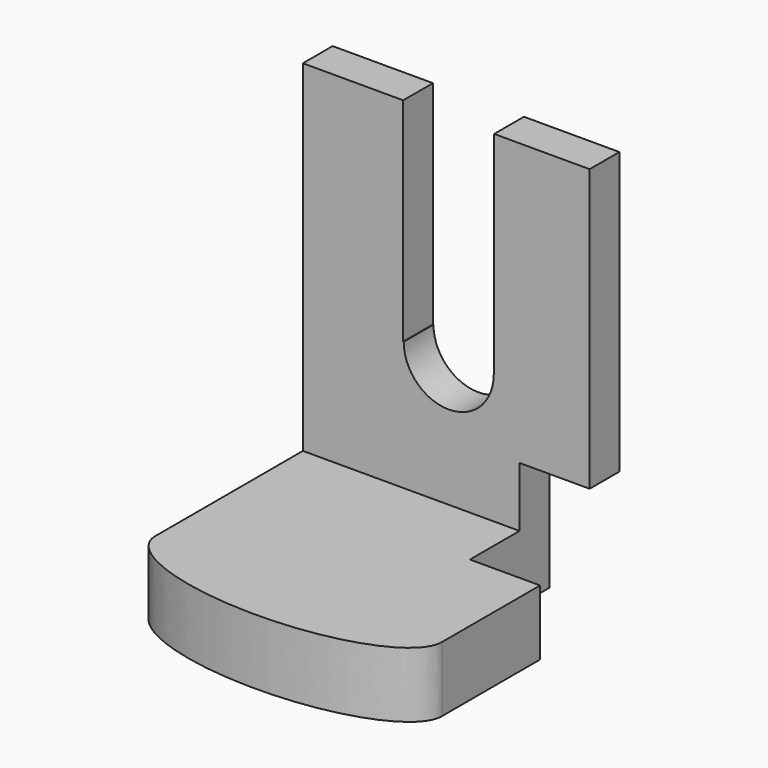
from build123d import *

# Parameters (mm, degrees)
F0_W      = 111.6153746843
F0_H      = 86.3690413535
F1_DEPTH  = 25.4
F2_W      = 111.6153746843
F2_H      = 132.8332849503
F3_DEPTH  = 14.478
F5_DEPTH  = 25.4
F6_W      = 27.2912848741
F6_H      = 24.1202692242
F6_H_2    = 22.7464084773
F7_DEPTH  = 56.134
F8_W      = 27.2912848741
F8_H      = 23.3086437643
F9_DEPTH  = 25.4
F10_W     = 35.4191940278
F10_H     = 82.6842561364
F11_DEPTH = 25.4
F13_DEPTH = 25.4


with BuildPart() as f1:
    # F0 (on Top) → F1 (new body)
    with BuildSketch(Plane.XY):
        with Locations((2.0880438387, 18.9822074026)):
            Rectangle(F0_W, F0_H)
    extrude(amount=F1_DEPTH)

    # F2 (on face) → F3 (join)
    with BuildSketch(Plane(origin=(0, 62.1667280793, 0), x_dir=(-1, 0, 0), z_dir=(0, 1, 0))):
        with Locations((-2.0880438387, 91.8166424751)):
            Rectangle(F2_W, F2_H)
    extrude(amount=-F3_DEPTH)

    # F4 (on face) → F5 (join)
    with BuildSketch(Plane.XY.offset(25.4)):
        with BuildLine():
            add(Edge.make_bspline(
                [(-53.7196435034, -24.2023132741), (-53.7196435034, -45.4823012569), (2.0880438387, -45.4823012569), (57.8957311809, -45.4823012569), (57.8957311809, -24.2023132741)],
                knots=[3.1415926536, 3.1415926536, 3.1415926536, 4.7123889804, 4.7123889804, 6.2831853072, 6.2831853072, 6.2831853072], degree=2, weights=[1, 0.7071067812, 1, 0.7071067812, 1]))
            Line((57.8957311809, -24.2023132741), (-53.7196435034, -24.2023132741))
        make_face()
    extrude(amount=-F5_DEPTH)

    # F6 (on face) → F7 (cut)
    with BuildSketch(Plane.XY.offset(25.4)):
        with Locations((44.2500887439, 35.6285934672)):
            Rectangle(F6_W, F6_H)
        with Locations((44.2500887439, 59.061932318)):
            Rectangle(F6_W, F6_H_2)
    extrude(amount=-F7_DEPTH, mode=Mode.SUBTRACT)

    # F8 (on face) → F9 (cut)
    with BuildSketch(Plane.XZ.offset(-47.6887280793)):
        with Locations((44.2500887439, 37.0543218821)):
            Rectangle(F8_W, F8_H)
    extrude(amount=-F9_DEPTH, mode=Mode.SUBTRACT)

    # F10 (on face) → F11 (cut)
    with BuildSketch(Plane.XZ.offset(-47.6887280793)):
        with Locations((3.0291331932, 116.891156882)):
            Rectangle(F10_W, F10_H)
    extrude(amount=-F11_DEPTH, mode=Mode.SUBTRACT)

    # F12 (on face) → F13 (cut)
    with BuildSketch(Plane.XZ.offset(-47.6887280793)):
        with BuildLine():
            ThreePointArc((-14.4735330019, 75.5490288138), (3.0291331932, 58.0463626187), (20.5317993883, 75.5490288138))
            Line((20.5317993883, 75.5490288138), (-14.4735330019, 75.5490288138))
        make_face()
    extrude(amount=-F13_DEPTH, mode=Mode.SUBTRACT)


solid = f1.part
